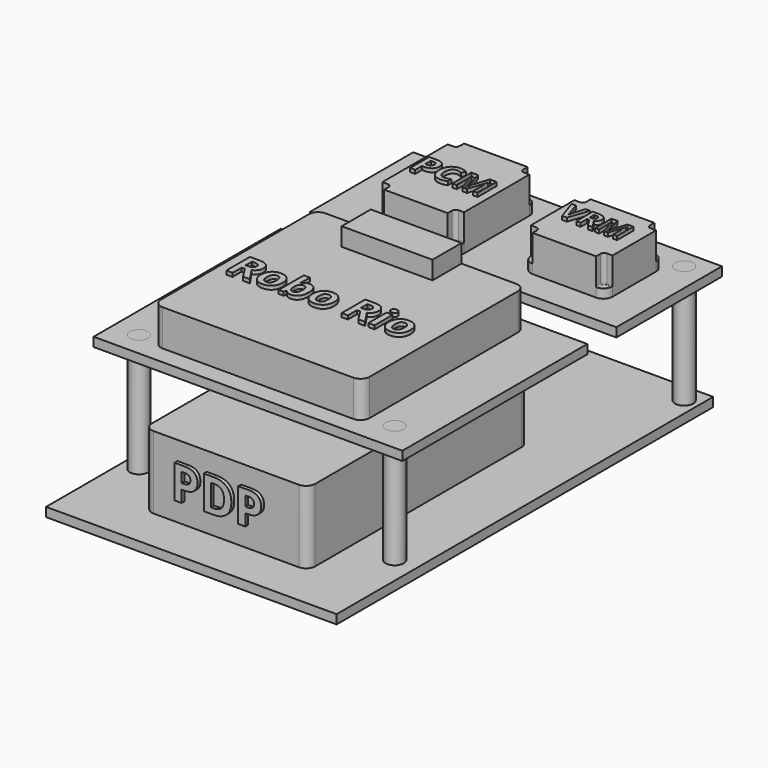
from build123d import *

# Parameters (mm, degrees)
F0_W          = 203.2
F0_H          = 254
F1_DEPTH      = 6.35
F3_DEPTH      = 50.8
F5_DEPTH      = 31.75
F7_DEPTH      = 304.292
F9_DEPTH      = 25.4
F10_W         = 63.5
F10_H         = 25.4
F11_DEPTH     = 12.7
F13_DEPTH     = 25.4
F15_DEPTH     = 25.4
F16_TEXT_SIZE = 32.5430184603
F17_DEPTH     = 2.54
F18_TEXT_SIZE = 28.892364567
F19_DEPTH     = 2.54
F20_TEXT_SIZE = 23.2710614845
F21_DEPTH     = 2.54
F22_TEXT_SIZE = 19.9523074765
F23_DEPTH     = 2.54
F24_R         = 6.35
F25_DEPTH     = 84.836
F26_R         = 6.35
F27_DEPTH     = 83.82
F28_DEPTH     = 75.184
F29_R         = 6.35
F30_DEPTH     = 85.09
F32_DEPTH     = 19.05
F33_R         = 0.6132102448
F35_DEPTH     = 19.05
F36_R         = 0.6096
F37_R         = 0.6096
F38_R         = 0.6096
F40_DEPTH     = 19.05
F41_R         = 0.6096
F42_R         = 0.6096
F43_R         = 0.6096
F44_R         = 0.6096
F45_W         = 25.4
F45_H         = 6.35
F46_DEPTH     = 82.55
F47_W         = 25.4
F47_H         = 6.35
F48_DEPTH     = 88.9


# Not quite as in the source:
# - Text() gives the source's letters only with a copy of the font that has no kerning and outlines rounded to 1/6400 em; it was checked with that copy


with BuildPart() as f1:
    # F0 (on Top) → F1 (new body)
    with BuildSketch(Plane.XY):
        with Locations((101.6, 127)):
            Rectangle(F0_W, F0_H)
    extrude(amount=F1_DEPTH)

    # F2 (on face) → F3 (join)
    with BuildSketch(Plane.XY.offset(6.35)):
        with BuildLine():
            Line((152.4, 223.52), (50.8, 223.52))
            ThreePointArc((50.8, 223.52), (46.3098719395, 221.6601280605), (44.45, 217.17))
            Line((44.45, 217.17), (44.45, 36.83))
            ThreePointArc((44.45, 36.83), (46.3098719395, 32.3398719395), (50.8, 30.48))
            Line((50.8, 30.48), (152.4, 30.48))
            ThreePointArc((152.4, 30.48), (156.8901280605, 32.3398719395), (158.75, 36.83))
            Line((158.75, 36.83), (158.75, 217.17))
            ThreePointArc((158.75, 217.17), (156.8901280605, 221.6601280605), (152.4, 223.52))
        make_face()
    extrude(amount=F3_DEPTH)

    # F4 (on face) → F5 (join)
    with BuildSketch(Plane.XY.offset(57.15)):
        with BuildLine():
            Line((-6.35, 49.53), (44.45, 49.53))
            Line((44.45, 49.53), (44.45, 217.17))
            ThreePointArc((44.45, 217.17), (46.3098719395, 221.6601280605), (50.8, 223.52))
            Line((50.8, 223.52), (152.4, 223.52))
            ThreePointArc((152.4, 223.52), (156.8901280605, 221.6601280605), (158.75, 217.17))
            Line((158.75, 217.17), (158.75, 49.53))
            Line((158.75, 49.53), (209.55, 49.53))
            Line((209.55, 49.53), (209.55, 328.93))
            Line((209.55, 328.93), (-6.35, 328.93))
            Line((-6.35, 328.93), (-6.35, 49.53))
        make_face()
        with BuildLine():
            Line((44.45, 49.53), (101.6, 49.53))
            Line((101.6, 49.53), (158.75, 49.53))
            Line((158.75, 49.53), (158.75, 217.17))
            ThreePointArc((158.75, 217.17), (156.8901280605, 221.6601280605), (152.4, 223.52))
            Line((152.4, 223.52), (50.8, 223.52))
            ThreePointArc((50.8, 223.52), (46.3098719395, 221.6601280605), (44.45, 217.17))
            Line((44.45, 217.17), (44.45, 49.53))
        make_face()
    extrude(amount=F5_DEPTH)

    # F6 (on face) → F7 (cut)
    with BuildSketch(Plane.XZ.offset(-49.53)):
        Polygon((-6.35, 82.55), (-6.35, 57.15), (44.45, 57.15), (158.75, 57.15), (209.55, 57.15), (209.55, 82.55), align=None)
    extrude(amount=-F7_DEPTH, mode=Mode.SUBTRACT)

    # F8 (on face) → F9 (join)
    with BuildSketch(Plane.XY.offset(88.9)):
        with BuildLine():
            ThreePointArc((25.4, 68.58), (27.2598719395, 64.0898719395), (31.75, 62.23))
            Line((31.75, 62.23), (165.1, 62.23))
            ThreePointArc((165.1, 62.23), (169.5901280605, 64.0898719395), (171.45, 68.58))
            Line((171.45, 68.58), (171.45, 198.12))
            ThreePointArc((171.45, 198.12), (169.5901280605, 202.6101280605), (165.1, 204.47))
            Line((165.1, 204.47), (31.75, 204.47))
            ThreePointArc((31.75, 204.47), (27.2598719395, 202.6101280605), (25.4, 198.12))
            Line((25.4, 198.12), (25.4, 68.58))
        make_face()
    extrude(amount=F9_DEPTH)

    # F10 (on face) → F11 (join)
    with BuildSketch(Plane.XY.offset(114.3)):
        with Locations((95.25, 191.77)):
            Rectangle(F10_W, F10_H)
    extrude(amount=F11_DEPTH)

    # F12 (on face) → F13 (join)
    with BuildSketch(Plane.XY.offset(88.9)):
        with BuildLine():
            ThreePointArc((185.3882565856, 301.5628566612), (183.5283846461, 306.0529847218), (179.0382565856, 307.9128566612))
            Line((179.0382565856, 307.9128566612), (134.5882565856, 307.9128566612))
            ThreePointArc((134.5882565856, 307.9128566612), (130.0981285251, 306.0529847218), (128.2382565856, 301.5628566612))
            Line((128.2382565856, 301.5628566612), (128.2382565856, 263.4628566612))
            ThreePointArc((128.2382565856, 263.4628566612), (130.0981285251, 258.9727286007), (134.5882565856, 257.1128566612))
            Line((134.5882565856, 257.1128566612), (179.0382565856, 257.1128566612))
            ThreePointArc((179.0382565856, 257.1128566612), (183.5283846461, 258.9727286007), (185.3882565856, 263.4628566612))
            Line((185.3882565856, 263.4628566612), (185.3882565856, 301.5628566612))
        make_face()
    extrude(amount=F13_DEPTH)

    # F14 (on face) → F15 (join)
    with BuildSketch(Plane.XY.offset(88.9)):
        with BuildLine():
            Line((83.7882565856, 316.23), (39.3382565856, 316.23))
            ThreePointArc((39.3382565856, 316.23), (34.8481285251, 314.3701280605), (32.9882565856, 309.88))
            Line((32.9882565856, 309.88), (32.9882565856, 252.73))
            ThreePointArc((32.9882565856, 252.73), (34.8481285251, 248.2398719395), (39.3382565856, 246.38))
            Line((39.3382565856, 246.38), (83.7882565856, 246.38))
            ThreePointArc((83.7882565856, 246.38), (88.2783846461, 248.2398719395), (90.1382565856, 252.73))
            Line((90.1382565856, 252.73), (90.1382565856, 309.88))
            ThreePointArc((90.1382565856, 309.88), (88.2783846461, 314.3701280605), (83.7882565856, 316.23))
        make_face()
    extrude(amount=F15_DEPTH)

    # F16 (on face) → F17 (join)
    with BuildSketch(Plane.XZ.offset(-30.48)):
        with Locations((64.5802021027, 20.895473659)):
            Text('PDP', F16_TEXT_SIZE, font='Open Sans', font_style=FontStyle.BOLD, text_align=(TextAlign.LEFT, TextAlign.BOTTOM))
    extrude(amount=F17_DEPTH)

    # F18 (on face) → F19 (join)
    with BuildSketch(Plane.XY.offset(114.3)):
        with Locations((32.2411602911, 114.0483026377)):
            Text('Robo Rio', F18_TEXT_SIZE, font='Open Sans', font_style=FontStyle.BOLD, text_align=(TextAlign.LEFT, TextAlign.BOTTOM))
    extrude(amount=F19_DEPTH)

    # F20 (on face) → F21 (join)
    with BuildSketch(Plane.XY.offset(114.3)):
        with Locations((35.3746600777, 271.4720301385)):
            Text('PCM', F20_TEXT_SIZE, font='Open Sans', font_style=FontStyle.BOLD, text_align=(TextAlign.LEFT, TextAlign.BOTTOM))
    extrude(amount=F21_DEPTH)

    # F22 (on face) → F23 (join)
    with BuildSketch(Plane.XY.offset(114.3)):
        with Locations((132.8552608285, 279.1300587311)):
            Text('VRM', F22_TEXT_SIZE, font='Open Sans', font_style=FontStyle.BOLD, text_align=(TextAlign.LEFT, TextAlign.BOTTOM))
    extrude(amount=F23_DEPTH)

    # F28 (add): a face of the model
    f28_faces = [f1.faces().sort_by_distance(p)[0] for p in [
        (101.6, 254, 3.175),
    ]]
    extrude(f28_faces, amount=F28_DEPTH)

    # F31 (on face) → F32 (cut)
    with BuildSketch(Plane.XY.offset(114.3)):
        with BuildLine():
            Line((179.0382565856, 260.9228566612), (179.0382565856, 257.1128566612))
            ThreePointArc((179.0382565856, 257.1128566612), (183.5283846461, 258.9727286007), (185.3882565856, 263.4628566612))
            Line((185.3882565856, 263.4628566612), (181.5782565856, 263.4628566612))
            ThreePointArc((181.5782565856, 263.4628566612), (179.7822053614, 262.7189078854), (179.0382565856, 260.9228566612))
        make_face()
    extrude(amount=-F32_DEPTH, mode=Mode.SUBTRACT)

    # F33
    f33_edges = [f1.edges().sort_by_distance(p)[0] for p in [
        (179.038257, 259.017857, 95.25),
        (183.483257, 263.462857, 95.25),
    ]]
    fillet(f33_edges, radius=F33_R)

    # F34 (on face) → F35 (cut)
    with BuildSketch(Plane.XY.offset(114.3)):
        with BuildLine():
            Line((132.0482565856, 263.4628566612), (128.2382565856, 263.4628566612))
            ThreePointArc((128.2382565856, 263.4628566612), (130.0981285251, 258.9727286007), (134.5882565856, 257.1128566612))
            Line((134.5882565856, 257.1128566612), (134.5882565856, 260.9228566612))
            ThreePointArc((134.5882565856, 260.9228566612), (133.8443078098, 262.7189078854), (132.0482565856, 263.4628566612))
        make_face()
        with BuildLine():
            ThreePointArc((134.5882565856, 307.9128566612), (130.0981285251, 306.0529847218), (128.2382565856, 301.5628566612))
            Line((128.2382565856, 301.5628566612), (132.0482565856, 301.5628566612))
            ThreePointArc((132.0482565856, 301.5628566612), (133.8443078098, 302.306805437), (134.5882565856, 304.1028566612))
            Line((134.5882565856, 304.1028566612), (134.5882565856, 307.9128566612))
        make_face()
        with BuildLine():
            ThreePointArc((185.3882565856, 301.5628566612), (183.5283846461, 306.0529847218), (179.0382565856, 307.9128566612))
            Line((179.0382565856, 307.9128566612), (179.0382565856, 304.1028566612))
            ThreePointArc((179.0382565856, 304.1028566612), (179.7822053614, 302.306805437), (181.5782565856, 301.5628566612))
            Line((181.5782565856, 301.5628566612), (185.3882565856, 301.5628566612))
        make_face()
    extrude(amount=-F35_DEPTH, mode=Mode.SUBTRACT)

    # F36
    f36_edges = [f1.edges().sort_by_distance(p)[0] for p in [
        (130.143257, 263.462857, 95.25),
        (134.588257, 259.017857, 95.25),
    ]]
    fillet(f36_edges, radius=F36_R)

    # F37
    f37_edges = [f1.edges().sort_by_distance(p)[0] for p in [
        (134.588257, 306.007857, 95.25),
        (130.143257, 301.562857, 95.25),
    ]]
    fillet(f37_edges, radius=F37_R)

    # F38
    f38_edges = [f1.edges().sort_by_distance(p)[0] for p in [
        (183.483257, 301.562857, 95.25),
        (179.038257, 306.007857, 95.25),
    ]]
    fillet(f38_edges, radius=F38_R)

    # F39 (on face) → F40 (cut)
    with BuildSketch(Plane.XY.offset(114.3)):
        with BuildLine():
            ThreePointArc((83.7882565856, 246.38), (88.2783846461, 248.2398719395), (90.1382565856, 252.73))
            Line((90.1382565856, 252.73), (86.3282565856, 252.73))
            ThreePointArc((86.3282565856, 252.73), (84.5322053614, 251.9860512242), (83.7882565856, 250.19))
            Line((83.7882565856, 250.19), (83.7882565856, 246.38))
        make_face()
        with BuildLine():
            Line((36.7982565856, 252.73), (32.9882565856, 252.73))
            ThreePointArc((32.9882565856, 252.73), (34.8481285251, 248.2398719395), (39.3382565856, 246.38))
            Line((39.3382565856, 246.38), (39.3382565856, 250.19))
            ThreePointArc((39.3382565856, 250.19), (38.5943078098, 251.9860512242), (36.7982565856, 252.73))
        make_face()
        with BuildLine():
            Line((39.3382565856, 312.42), (39.3382565856, 316.23))
            ThreePointArc((39.3382565856, 316.23), (34.8481285251, 314.3701280605), (32.9882565856, 309.88))
            Line((32.9882565856, 309.88), (36.7982565856, 309.88))
            ThreePointArc((36.7982565856, 309.88), (38.5943078098, 310.6239487758), (39.3382565856, 312.42))
        make_face()
        with BuildLine():
            ThreePointArc((90.1382565856, 309.88), (88.2783846461, 314.3701280605), (83.7882565856, 316.23))
            Line((83.7882565856, 316.23), (83.7882565856, 312.42))
            ThreePointArc((83.7882565856, 312.42), (84.5322053614, 310.6239487758), (86.3282565856, 309.88))
            Line((86.3282565856, 309.88), (90.1382565856, 309.88))
        make_face()
    extrude(amount=-F40_DEPTH, mode=Mode.SUBTRACT)

    # F41
    f41_edges = [f1.edges().sort_by_distance(p)[0] for p in [
        (39.338257, 314.325, 95.25),
        (34.893257, 309.88, 95.25),
    ]]
    fillet(f41_edges, radius=F41_R)

    # F42
    f42_edges = [f1.edges().sort_by_distance(p)[0] for p in [
        (88.233257, 309.88, 95.25),
        (83.788257, 314.325, 95.25),
    ]]
    fillet(f42_edges, radius=F42_R)

    # F43
    f43_edges = [f1.edges().sort_by_distance(p)[0] for p in [
        (83.788257, 248.285, 95.25),
        (84.532205, 251.986051, 95.25),
        (88.233257, 252.73, 95.25),
    ]]
    fillet(f43_edges, radius=F43_R)

    # F44
    f44_edges = [f1.edges().sort_by_distance(p)[0] for p in [
        (34.893257, 252.73, 95.25),
        (39.338257, 248.285, 95.25),
    ]]
    fillet(f44_edges, radius=F44_R)

    # F45 (on face) → F46 (cut)
    with BuildSketch(Plane.YZ.offset(209.55)):
        with Locations((223.9605273724, 85.725)):
            Rectangle(F45_W, F45_H)
    extrude(amount=-F46_DEPTH, mode=Mode.SUBTRACT)

    # F47 (on face) → F48 (cut)
    with BuildSketch(Plane(origin=(-6.35, 0, 0), x_dir=(0, -1, 0), z_dir=(-1, 0, 0))):
        with Locations((-225.8777235031, 85.725)):
            Rectangle(F47_W, F47_H)
    extrude(amount=-F48_DEPTH, mode=Mode.SUBTRACT)


with BuildPart() as f25:
    # F24 (on face) → F25 (new body)
    with BuildSketch(Plane.XY.offset(88.9)):
        with Locations((187.9368573427, 69.8686167598)):
            Circle(F24_R)
    extrude(amount=-F25_DEPTH)


with BuildPart() as f27:
    # F26 (on face) → F27 (new body)
    with BuildSketch(Plane.XY.offset(88.9)):
        with Locations((11.6681223735, 66.6432455182)):
            Circle(F26_R)
    extrude(amount=-F27_DEPTH)


with BuildPart() as f30:
    # F29 (on face) → F30 (new body)
    with BuildSketch(Plane.XY.offset(88.9)):
        with Locations((13.1987297865, 312.5341948569)):
            Circle(F29_R)
    extrude(amount=-F30_DEPTH)


with BuildPart() as f30b:
    # F29 (on face) → F30, piece 2 (new body)
    with BuildSketch(Plane.XY.offset(88.9)):
        with Locations((193.4075358604, 316.0814441275)):
            Circle(F29_R)
    extrude(amount=-F30_DEPTH)


solid = Compound([f1.part, f25.part, f27.part, f30.part, f30b.part])
